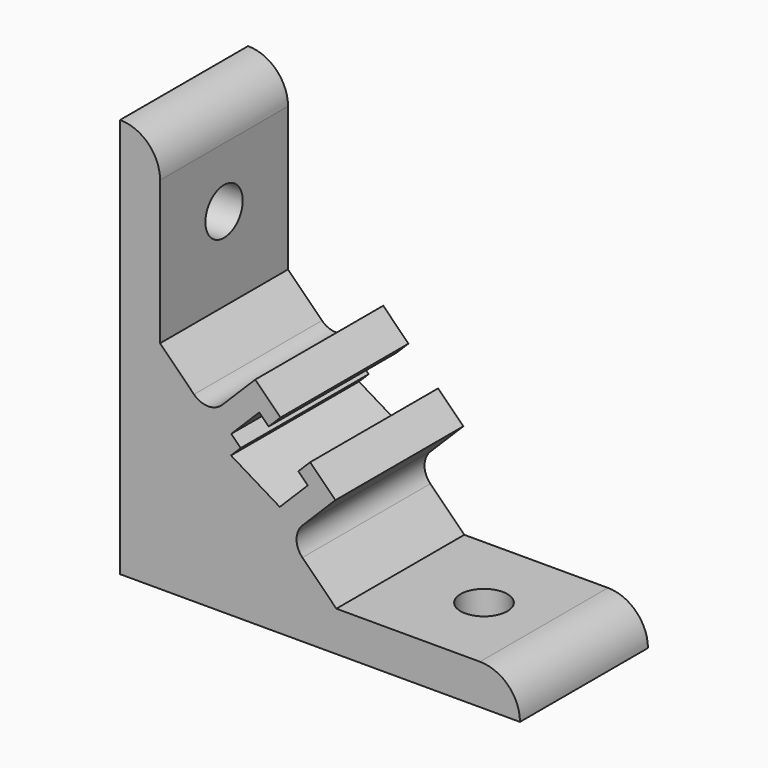
from build123d import *

# Parameters (mm, degrees)
F1_DEPTH = 24
F2_R     = 3.5
F3_DEPTH = 6
F4_R     = 3.5
F5_DEPTH = 6


# Not quite as in the source:
# - ends of sketch curves that miss each other by under 0.0002 mm in the source are joined


with BuildPart() as f1:
    # F0 (on Front) → F1 (new body)
    with BuildSketch(Plane.XZ):
        with BuildLine():
            Line((5.999886, 45.000227), (-0.000114, 45.000227))
            Line((-0.000114, 45.000227), (-0.000114, 0.000227))
            Line((-0.000114, 0.000227), (44.999886, 0.000227))
            Line((44.999886, 0.000227), (44.999886, 6.000227))
            Line((44.999886, 6.000227), (32.449634, 6.000227))
            Line((32.449634, 6.000227), (27.356487, 11.093373))
            ThreePointArc((27.356487, 11.093373), (26.477808, 13.214693), (27.3564876564, 15.3360133436))
            Line((27.3564876564, 15.3360133436), (32.306235, 20.285761))
            Line((32.306235, 20.285761), (28.523214, 24.068783))
            Line((28.523214, 24.068783), (26.755447, 22.301016))
            Line((26.755447, 22.301016), (28.16966, 20.886802))
            Line((28.16966, 20.886802), (23.960753, 16.677895))
            Line((23.960753, 16.677895), (16.64382, 21.098934))
            Line((16.64382, 21.098934), (18.091767, 22.546881))
            Line((18.091767, 22.546881), (16.677553, 23.961095))
            Line((16.677553, 23.961095), (20.88646, 28.170002))
            Line((20.88646, 28.170002), (22.300674, 26.755788))
            Line((22.300674, 26.755788), (24.068441, 28.523555))
            Line((24.068441, 28.523555), (20.28542, 32.306577))
            Line((20.28542, 32.306577), (15.335672, 27.356829))
            ThreePointArc((15.335672, 27.356829), (13.2143523536, 26.47815), (11.0930316564, 27.3568296564))
            Line((11.0930316564, 27.3568296564), (5.999886, 32.449975))
            Line((5.999886, 32.449975), (5.999886, 45.000227))
        make_face()
        with BuildLine():
            ThreePointArc((4.499886, 4.000227), (4.1463326094, 4.1466736094), (3.999886, 4.500227))
            Line((3.999886, 4.500227), (3.999886, 29.000227))
            ThreePointArc((3.999886, 29.000227), (4.3085446105, 29.4621669016), (4.8534398906, 29.3537798906))
            Line((4.8534398906, 29.3537798906), (13.567905, 20.639315))
            Line((13.567905, 20.639315), (11.243789, 18.315199))
            ThreePointArc((11.243789, 18.315199), (10.3880809238, 17.170688427), (9.8910739732, 15.8308650058))
            Line((9.8910739732, 15.8308650058), (11.753138, 13.968801))
            Line((11.753138, 13.968801), (12.364509, 14.132617))
            ThreePointArc((12.364509, 14.132617), (16.54708952, 16.547432386), (14.1322760675, 12.364850252))
            Line((14.1322760675, 12.364850252), (13.968459, 11.75348))
            Line((13.968459, 11.75348), (15.830523, 9.891416))
            ThreePointArc((15.830523, 9.891416), (17.1703461165, 10.3884227548), (18.3148569059, 11.2441310941))
            Line((18.3148569059, 11.2441310941), (20.638973, 13.568247))
            Line((20.638973, 13.568247), (29.353439, 4.853781))
            ThreePointArc((29.353439, 4.853781), (29.461825631, 4.3088849572), (28.999886, 4.000227))
            Line((28.999886, 4.000227), (4.499886, 4.000227))
        make_face(mode=Mode.SUBTRACT)
        with BuildLine():
            Line((3.999886, 29.000227), (3.999886, 4.500227))
            ThreePointArc((3.999886, 4.500227), (4.1463326094, 4.1466736094), (4.499886, 4.000227))
            Line((4.499886, 4.000227), (28.999886, 4.000227))
            ThreePointArc((28.999886, 4.000227), (29.461825631, 4.3088849572), (29.3534398906, 4.8537798906))
            Line((29.3534398906, 4.8537798906), (20.638973, 13.568247))
            Line((20.638973, 13.568247), (18.314857, 11.244131))
            ThreePointArc((18.314857, 11.244131), (17.1703461165, 10.3884227548), (15.8305230058, 9.8914159732))
            Line((15.8305230058, 9.8914159732), (13.968459, 11.75348))
            Line((13.968459, 11.75348), (14.132276, 12.36485))
            ThreePointArc((14.132276, 12.36485), (16.54708952, 16.547432386), (12.364508569, 14.1326168845))
            Line((12.364508569, 14.1326168845), (11.753138, 13.968801))
            Line((11.753138, 13.968801), (9.891074, 15.830865))
            ThreePointArc((9.891074, 15.830865), (10.3880809238, 17.170688427), (11.2437895941, 18.3151994059))
            Line((11.2437895941, 18.3151994059), (13.567905, 20.639315))
            Line((13.567905, 20.639315), (4.853439, 29.353781))
            ThreePointArc((4.853439, 29.353781), (4.3085446105, 29.4621669016), (3.999886, 29.000227))
        make_face()
        with BuildLine():
            ThreePointArc((5.999886, 54.000227), (4.2425266871, 58.2428676871), (-0.000114, 60.000227))
            Line((-0.000114, 60.000227), (-0.000114, 45.000227))
            Line((-0.000114, 45.000227), (5.999886, 45.000227))
            Line((5.999886, 45.000227), (5.999886, 54.000227))
        make_face()
        with BuildLine():
            Line((44.999886, 6.000227), (44.999886, 0.000227))
            Line((44.999886, 0.000227), (59.999886, 0.000227))
            ThreePointArc((59.999886, 0.000227), (58.2425266871, 4.2428676871), (53.999886, 6.000227))
            Line((53.999886, 6.000227), (44.999886, 6.000227))
        make_face()
    extrude(amount=-F1_DEPTH)

    # F2 (on face) → F3 (cut)
    with BuildSketch(Plane(origin=(-0.000114, 0, 0), x_dir=(0, -1, 0), z_dir=(-1, 0, 0))):
        with Locations((-12, 45.000227)):
            Circle(F2_R)
    extrude(amount=-F3_DEPTH, mode=Mode.SUBTRACT)

    # F4 (on face) → F5 (cut)
    with BuildSketch(Plane(origin=(0, 0, 0.000227), x_dir=(1, 0, 0), z_dir=(0, 0, -1))):
        with Locations((44.999886, -12)):
            Circle(F4_R)
    extrude(amount=-F5_DEPTH, mode=Mode.SUBTRACT)


solid = f1.part
